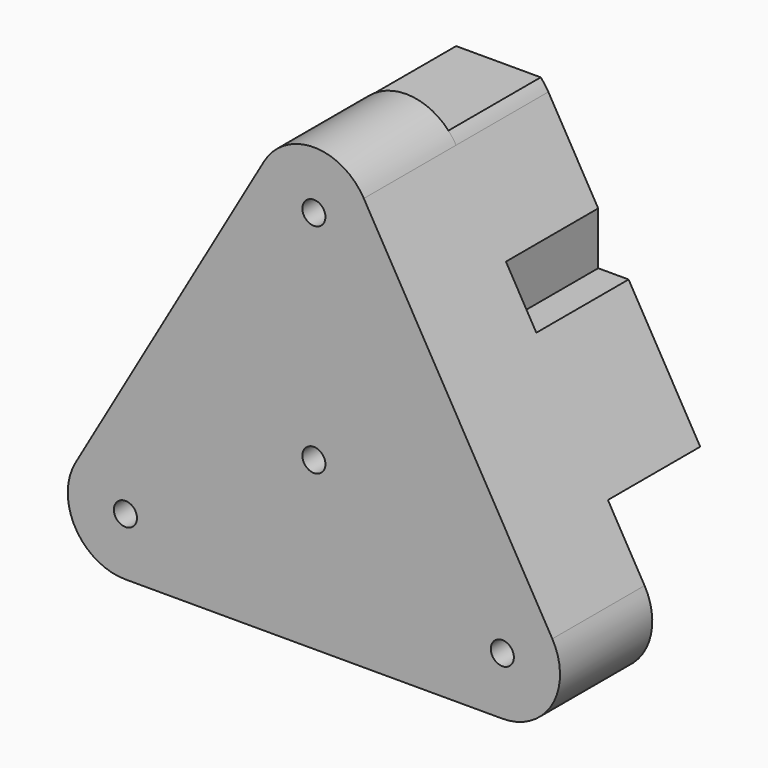
from build123d import *

# Parameters (mm, degrees)
F1_DEPTH = 10
F3_D     = 2
F3_DEPTH = 12
F3_TIP   = 0.600860619
F4_R     = 1
F5_DEPTH = 10


with BuildPart() as f1:
    # F0 (on Front) → F1 (new body)
    with BuildSketch(Plane.XZ):
        with BuildLine():
            Line((-4.3301270189, 21.3675134595), (-20.6698729811, -6.9337567297))
            ThreePointArc((-20.6698729811, -6.9337567297), (-20.6698729811, -11.9337567297), (-16.3397459622, -14.4337567297))
            Line((-16.3397459622, -14.4337567297), (16.3397459622, -14.4337567297))
            ThreePointArc((16.3397459622, -14.4337567297), (20.6698729811, -11.9337567297), (20.6698729811, -6.9337567297))
            Line((20.6698729811, -6.9337567297), (4.3301270189, 21.3675134595))
            ThreePointArc((4.3301270189, 21.3675134595), (0, 23.8675134595), (-4.3301270189, 21.3675134595))
        make_face()
    extrude(amount=F1_DEPTH)

    # F3
    with Locations(Plane.XZ.offset(10)):
        with Locations((0, 18.8675134595), (0, 0), (16.3397459622, -9.4337567297), (-16.3397459622, -9.4337567297)):
            Hole(F3_D / 2, depth=F3_DEPTH)
            with Locations((0, 0, -(F3_DEPTH + F3_TIP / 2))):  # 118° drill point
                Cone(0, F3_D / 2, F3_TIP, mode=Mode.SUBTRACT)

    # F4 (on face) → F5 (join)
    with BuildSketch(Plane(origin=(0, 0, 0), x_dir=(-1, 0, 0), z_dir=(0, 1, 0))):
        with BuildLine():
            Line((-11.2879311067, 9.3162432703), (-17.4944465005, -1.4337567297))
            Line((-17.4944465005, -1.4337567297), (12.25, -1.4337567297))
            Line((12.25, -1.4337567297), (12.25, -14.4337567297))
            Line((12.25, -14.4337567297), (16.3397459622, -14.4337567297))
            ThreePointArc((16.3397459622, -14.4337567297), (20.6698729811, -11.9337567297), (20.6698729811, -6.9337567297))
            Line((20.6698729811, -6.9337567297), (4.3301270189, 21.3675134595))
            ThreePointArc((4.3301270189, 21.3675134595), (4.0238527859, 21.8354435053), (3.6672381533, 22.2662432703))
            Line((3.6672381533, 22.2662432703), (-3.6672381533, 22.2662432703))
            ThreePointArc((-3.6672381533, 22.2662432703), (-4.0238527859, 21.8354435053), (-4.3301270189, 21.3675134595))
            Line((-4.3301270189, 21.3675134595), (-8.65, 13.885273974))
            Line((-8.65, 13.885273974), (-8.65, 9.3162432703))
            Line((-8.65, 9.3162432703), (-11.2879311067, 9.3162432703))
        make_face()
        with Locations((16.3397459622, -9.4337567297)):
            Circle(F4_R, mode=Mode.SUBTRACT)
        Circle(F4_R, mode=Mode.SUBTRACT)
        with Locations((0, 18.8675134595)):
            Circle(F4_R, mode=Mode.SUBTRACT)
        with Locations((16.3397459622, -9.4337567297)):
            Circle(F4_R)
        Circle(F4_R)
        with Locations((0, 18.8675134595)):
            Circle(F4_R)
    extrude(amount=F5_DEPTH)


solid = f1.part
